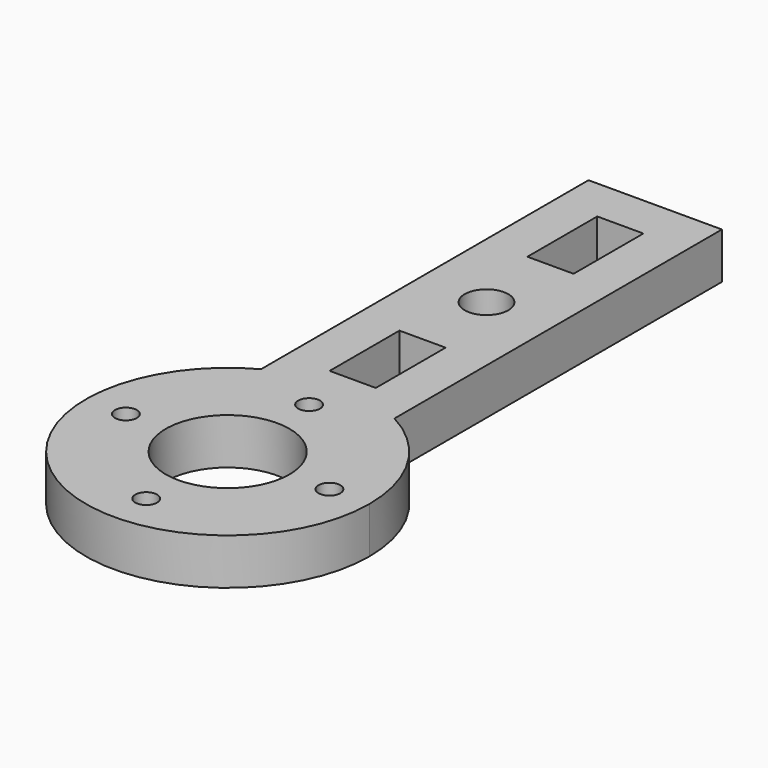
from build123d import *

# Parameters (mm, degrees)
F0_W     = 3.175
F0_H     = 6
F0_R     = 0.75
F1_DEPTH = 3.175


# Not quite as in the source:
# - a length typed as a fraction of an inch, garbled in the dataset ("3 / 203.2 mm" for 3/8 in), is restored


with BuildPart() as f1:
    # F0 (on Top) → F1 (new body)
    with BuildSketch(Plane.XY):
        with BuildLine():
            ThreePointArc((-25.3152321216, 19.8451589555), (-20.7277321216, 20.9918256626), (-16.1402321216, 19.8451589555))
            Line((-16.1402321216, 19.8451589555), (-16.1402321216, 47.9918256626))
            Line((-16.1402321216, 47.9918256626), (-25.3152321216, 47.9918256626))
            Line((-25.3152321216, 47.9918256626), (-25.3152321216, 19.8451589555))
        make_face()
        with Locations((-20.7277321216, 24.9918256626)):
            Rectangle(F0_W, F0_H, mode=Mode.SUBTRACT)
        with BuildLine():
            ThreePointArc((-22.2277321216, 33.4918256626), (-20.7277321216, 34.9918256626), (-19.2277321216, 33.4918256626))
            ThreePointArc((-19.2277321216, 33.4918256626), (-20.7277321216, 31.9918256626), (-22.2277321216, 33.4918256626))
        make_face(mode=Mode.SUBTRACT)
        with Locations((-20.7277321216, 41.9918256626)):
            Rectangle(F0_W, F0_H, mode=Mode.SUBTRACT)
        with BuildLine():
            ThreePointArc((-25.3152321216, 19.8451589555), (-25.744423013, 2.8814840128), (-10.9777321216, 11.2418256626))
            ThreePointArc((-10.9777321216, 11.2418256626), (-12.3673904719, 16.258516554), (-16.1402321216, 19.8451589555))
            ThreePointArc((-16.1402321216, 19.8451589555), (-20.7277321216, 20.9918256626), (-25.3152321216, 19.8451589555))
        make_face()
        with Locations((-27.7277321216, 11.2418256626)):
            Circle(F0_R, mode=Mode.SUBTRACT)
        with Locations((-20.7277321216, 4.2418256626)):
            Circle(F0_R, mode=Mode.SUBTRACT)
        with BuildLine():
            ThreePointArc((-20.7277321216, 6.9918256626), (-23.7329359416, 14.2470294826), (-16.4777321216, 11.2418256626))
            ThreePointArc((-16.4777321216, 11.2418256626), (-17.7225283015, 8.2366218425), (-20.7277321216, 6.9918256626))
        make_face(mode=Mode.SUBTRACT)
        with Locations((-13.7277321216, 11.2418256626)):
            Circle(F0_R, mode=Mode.SUBTRACT)
        with Locations((-20.7277321216, 18.2418256626)):
            Circle(F0_R, mode=Mode.SUBTRACT)
    extrude(amount=F1_DEPTH)


solid = f1.part
